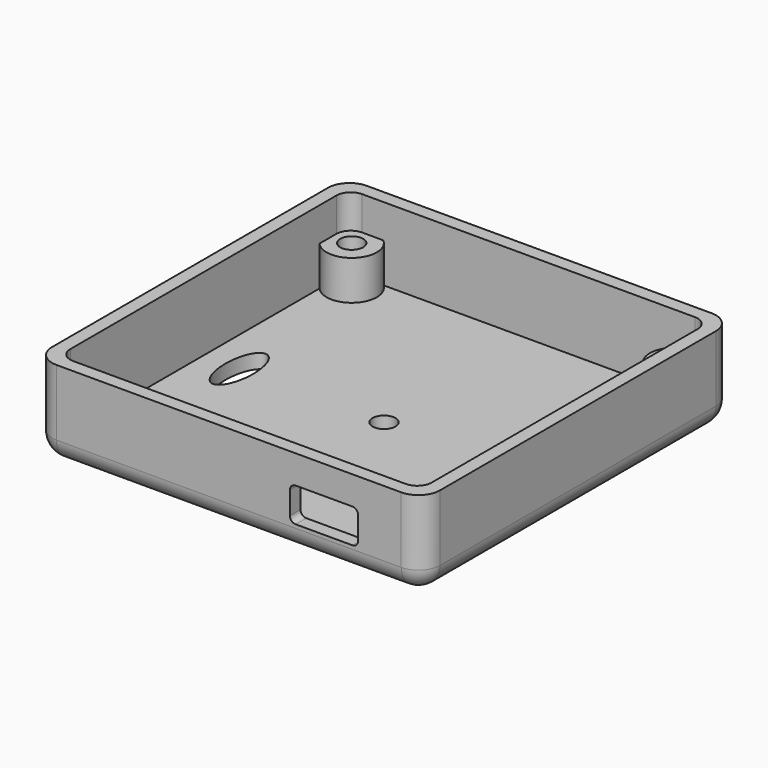
from build123d import *

# Parameters (mm, degrees)
F0_W          = 54
F0_H          = 54
F1_DEPTH      = 2
F2_W          = 54
F2_H          = 54
F2_W_2        = 50.3
F2_H_2        = 50.3
F3_DEPTH      = 10.2
F4_R          = 3.5
F5_DEPTH      = 5.5
F6_R          = 1.6
F7_DEPTH      = 25
F8_W          = 9.5
F8_H          = 4.75
F9_DEPTH      = 25
F11_DEPTH     = 25
F12_T1_DEPTH  = 48
F12_T3_DEPTH  = 48
F12_T5_DEPTH  = 16.7
F12_S9_W      = 3
F12_S9_H      = 3
F12_T10_DEPTH = 3
F12_S15_W     = 3
F12_S15_H     = 3
F12_T16_DEPTH = 3
F12_S21_W     = 3
F12_S21_H     = 3
F12_T22_DEPTH = 3
F12_S27_W     = 3
F12_S27_H     = 3
F12_T28_DEPTH = 3
F13_R         = 3
F14_DEPTH     = 2.5
F15_R         = 0.8
F16_R         = 2


# Not quite as in the source:
# - a fillet or chamfer that OpenCascade refuses, or shapes differently, is made with other operations: its cross-section is extruded or revolved along the edge and cut away or added


with BuildPart() as f1:
    # F0 (on Top) → F1 (new body)
    with BuildSketch(Plane.XY):
        Rectangle(F0_W, F0_H)
    extrude(amount=F1_DEPTH)

    # F2 (on face) → F3 (join)
    with BuildSketch(Plane.XY.offset(2)):
        Rectangle(F2_W, F2_H)
        Rectangle(F2_W_2, F2_H_2, mode=Mode.SUBTRACT)
    extrude(amount=F3_DEPTH)

    # F4 (on face) → F5 (join)
    with BuildSketch(Plane.XY.offset(2)):
        with Locations((-22.5, 22.5)):
            Circle(F4_R)
        with Locations((22.5, 22.5)):
            Circle(F4_R)
        with Locations((22.5, -22.5)):
            Circle(F4_R)
        with Locations((-22.5, -22.5)):
            Circle(F4_R)
    extrude(amount=F5_DEPTH)

    # F6 (on face) → F7 (cut)
    with BuildSketch(Plane(origin=(0, 0, 0), x_dir=(1, 0, 0), z_dir=(0, 0, -1))):
        with Locations((-22.5, 22.5)):
            Circle(F6_R)
        with Locations((22.5, 22.5)):
            Circle(F6_R)
        with Locations((22.5, -22.5)):
            Circle(F6_R)
        with Locations((-22.5, -22.5)):
            Circle(F6_R)
        Circle(F6_R)
    extrude(amount=-F7_DEPTH, mode=Mode.SUBTRACT)

    # F8 (on face) → F9 (cut)
    with BuildSketch(Plane.XZ.offset(27)):
        with Locations((13.25, 5.875)):
            Rectangle(F8_W, F8_H)
    extrude(amount=-F9_DEPTH, mode=Mode.SUBTRACT)

    # F10 (on face) → F11 (cut)
    with BuildSketch(Plane.XY.offset(2)):
        with BuildLine():
            add(Edge.make_bspline(
                [(-20.15, 4.5483106502), (-23.5056844979, 4.5483106502), (-21.827842249, -2.2741553251), (-20.15, -9.0966213004), (-18.472157751, -2.2741553251), (-16.7943155021, 4.5483106502), (-20.15, 4.5483106502)],
                knots=[0, 0, 0, 2.0943951024, 2.0943951024, 4.1887902048, 4.1887902048, 6.2831853072, 6.2831853072, 6.2831853072], degree=2, weights=[1, 0.5, 1, 0.5, 1, 0.5, 1]))
        make_face()
    extrude(amount=-F11_DEPTH, mode=Mode.SUBTRACT)

    # F12: fillet of radius 3 on 8 edges, made by hand

    # F12_s2 → F12_t1 (cut)
    with BuildSketch(Plane.YZ.offset(-24)):
        with BuildLine():
            ThreePointArc((-24, 0), (-26.1213203436, 0.8786796564), (-27, 3))
            Line((-27, 3), (-27, 0))
            Line((-27, 0), (-24, 0))
        make_face()
        with BuildLine():
            ThreePointArc((27, 3), (26.1213203436, 0.8786796564), (24, 0))
            Line((24, 0), (27, 0))
            Line((27, 0), (27, 3))
        make_face()
    extrude(amount=F12_T1_DEPTH, mode=Mode.SUBTRACT)

    # F12_s4 → F12_t3 (cut)
    with BuildSketch(Plane.XZ.offset(-24)):
        with BuildLine():
            ThreePointArc((-27, 3), (-26.1213203436, 0.8786796564), (-24, 0))
            Line((-24, 0), (-27, 0))
            Line((-27, 0), (-27, 3))
        make_face()
        with BuildLine():
            ThreePointArc((27, 3), (26.1213203436, 0.8786796564), (24, 0))
            Line((24, 0), (27, 0))
            Line((27, 0), (27, 3))
        make_face()
    extrude(amount=F12_T3_DEPTH, mode=Mode.SUBTRACT)

    # F12_s6 → F12_t5 (cut)
    with BuildSketch(Plane.XY.offset(3)):
        with BuildLine():
            ThreePointArc((27, -24), (26.1213203436, -26.1213203436), (24, -27))
            Line((24, -27), (27, -27))
            Line((27, -27), (27, -24))
        make_face()
        with BuildLine():
            ThreePointArc((-27, -24), (-26.1213203436, -26.1213203436), (-24, -27))
            Line((-24, -27), (-27, -27))
            Line((-27, -27), (-27, -24))
        make_face()
        with BuildLine():
            ThreePointArc((-24, 27), (-26.1213203436, 26.1213203436), (-27, 24))
            Line((-27, 24), (-27, 27))
            Line((-27, 27), (-24, 27))
        make_face()
        with BuildLine():
            ThreePointArc((24, 27), (26.1213203436, 26.1213203436), (27, 24))
            Line((27, 24), (27, 27))
            Line((27, 27), (24, 27))
        make_face()
    extrude(amount=F12_T5_DEPTH, mode=Mode.SUBTRACT)


with BuildPart() as f12_tool8:
    # F12_s9 → F12_t10 (new body)
    with BuildSketch(Plane.YZ.offset(-24)):
        with Locations((-25.5, 1.5)):
            Rectangle(F12_S9_W, F12_S9_H)
    extrude(amount=-F12_T10_DEPTH)

    # F12_s11 → F12_t12 (revolve, cut)
    with BuildSketch(Plane(origin=(-24, -24, 3), x_dir=(0, 0.7071067812, 0.7071067812), z_dir=(0, -0.7071067812, 0.7071067812))):
        with BuildLine():
            ThreePointArc((0, -3), (3, 0), (0, 3))
            Line((0, 3), (0, -3))
        make_face()
    revolve(axis=Axis((-24, -24, 3), (-1, 0, 0)), mode=Mode.SUBTRACT)


with BuildPart() as f1_1:
    add(f1.part)

    # F12_t7: cut F12_tool8
    add(f12_tool8.part, mode=Mode.SUBTRACT)


with BuildPart() as f12_tool14:
    # F12_s15 → F12_t16 (new body)
    with BuildSketch(Plane.YZ.offset(24)):
        with Locations((-25.5, 1.5)):
            Rectangle(F12_S15_W, F12_S15_H)
    extrude(amount=F12_T16_DEPTH)

    # F12_s17 → F12_t18 (revolve, cut)
    with BuildSketch(Plane(origin=(24, -24, 3), x_dir=(0, 0.7071067812, 0.7071067812), z_dir=(0, 0.7071067812, -0.7071067812))):
        with BuildLine():
            ThreePointArc((0, -3), (3, 0), (0, 3))
            Line((0, 3), (0, -3))
        make_face()
    revolve(axis=Axis((24, -24, 3), (1, 0, 0)), mode=Mode.SUBTRACT)


with BuildPart() as f1_2:
    add(f1_1.part)

    # F12_t13: cut F12_tool14
    add(f12_tool14.part, mode=Mode.SUBTRACT)


with BuildPart() as f12_tool20:
    # F12_s21 → F12_t22 (new body)
    with BuildSketch(Plane.XZ.offset(-24)):
        with Locations((-25.5, 1.5)):
            Rectangle(F12_S21_W, F12_S21_H)
    extrude(amount=-F12_T22_DEPTH)

    # F12_s23 → F12_t24 (revolve, cut)
    with BuildSketch(Plane(origin=(-24, 24, 3), x_dir=(0.7071067812, 0, 0.7071067812), z_dir=(-0.7071067812, 0, 0.7071067812))):
        with BuildLine():
            ThreePointArc((0, -3), (3, 0), (0, 3))
            Line((0, 3), (0, -3))
        make_face()
    revolve(axis=Axis((-24, 24, 3), (0, 1, 0)), mode=Mode.SUBTRACT)


with BuildPart() as f1_3:
    add(f1_2.part)

    # F12_t19: cut F12_tool20
    add(f12_tool20.part, mode=Mode.SUBTRACT)


with BuildPart() as f12_tool26:
    # F12_s27 → F12_t28 (new body)
    with BuildSketch(Plane.XZ.offset(-24)):
        with Locations((25.5, 1.5)):
            Rectangle(F12_S27_W, F12_S27_H)
    extrude(amount=-F12_T28_DEPTH)

    # F12_s29 → F12_t30 (revolve, cut)
    with BuildSketch(Plane(origin=(24, 24, 3), x_dir=(-0.7071067812, 0, 0.7071067812), z_dir=(-0.7071067812, 0, -0.7071067812))):
        with BuildLine():
            ThreePointArc((0, -3), (3, 0), (0, 3))
            Line((0, 3), (0, -3))
        make_face()
    revolve(axis=Axis((24, 24, 3), (0, 1, 0)), mode=Mode.SUBTRACT)


with BuildPart() as f1_4:
    add(f1_3.part)

    # F12_t25: cut F12_tool26
    add(f12_tool26.part, mode=Mode.SUBTRACT)

    # F13 (on face) → F14 (cut)
    with BuildSketch(Plane(origin=(0, 0, 0), x_dir=(1, 0, 0), z_dir=(0, 0, -1))):
        with Locations((-22.5, 22.5)):
            Circle(F13_R)
        with Locations((22.5, 22.5)):
            Circle(F13_R)
        with Locations((22.5, -22.5)):
            Circle(F13_R)
        with Locations((-22.5, -22.5)):
            Circle(F13_R)
    extrude(amount=-F14_DEPTH, mode=Mode.SUBTRACT)

    # F15
    f15_edges = [f1_4.edges().sort_by_distance(p)[0] for p in [
        (8.5, -26.075, 8.25),
        (8.5, -26.075, 3.5),
        (18, -26.075, 3.5),
        (18, -26.075, 8.25),
    ]]
    fillet(f15_edges, radius=F15_R)

    # F16
    f16_edges = [f1_4.edges().sort_by_distance(p)[0] for p in [
        (-25.15, 25.15, 7.1),
        (25.15, 25.15, 7.1),
        (-25.15, -25.15, 7.1),
        (25.15, -25.15, 7.1),
    ]]
    fillet(f16_edges, radius=F16_R)


solid = f1_4.part
